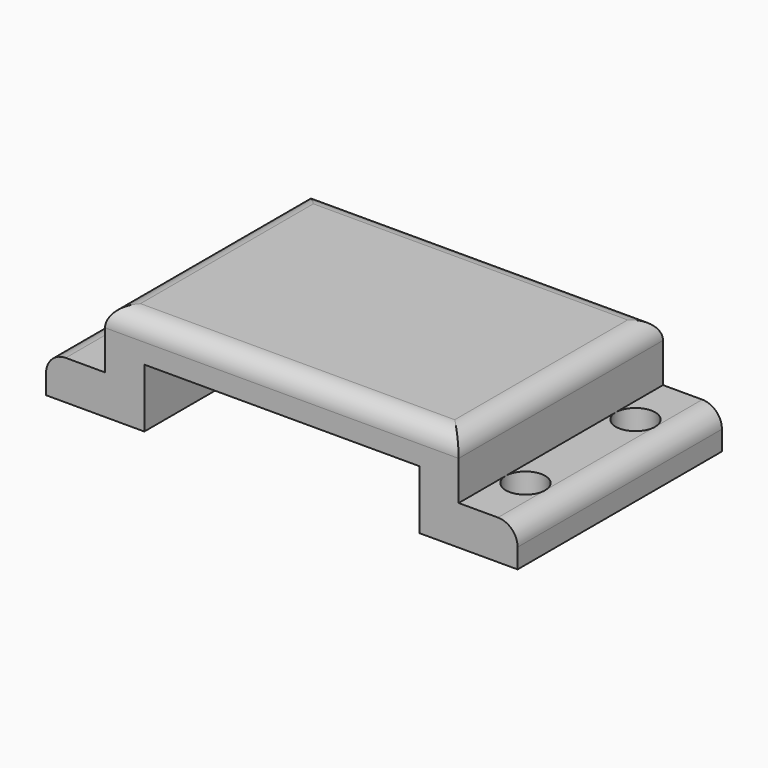
from build123d import *

# Parameters (mm, degrees)
F1_DEPTH = 13
F2_R     = 1
F3_R     = 1
F4_DEPTH = 25
F5_R     = 1
F6_DEPTH = 25


with BuildPart() as f1:
    # F0 (on Front) → F1 (new body)
    with BuildSketch(Plane.XZ):
        Polygon((-20.4238126724, 0), (-18.61380395, 0), (-15.4238126724, 0), (-15.4238126724, 3), (-1.4238126724, 3), (-1.4238126724, 0), (3.5761873276, 0), (3.5761873276, 2), (0.5761873276, 2), (0.5761873276, 5), (-17.4186695367, 5), (-17.4238126724, 2), (-20.4238126724, 2), align=None)
    extrude(amount=F1_DEPTH)

    # F2
    f2_edges = [f1.edges().sort_by_distance(p)[0] for p in [
        (-8.421241, 0, 5),
        (0.576187, -6.5, 5),
        (-17.41867, -6.5, 5),
        (-8.421241, -13, 5),
        (3.576187, -6.5, 2),
        (-20.423813, -6.5, 2),
    ]]
    fillet(f2_edges, radius=F2_R)

    # F3 (on face) → F4 (cut)
    with BuildSketch(Plane(origin=(0, 0, 0), x_dir=(1, 0, 0), z_dir=(0, 0, -1))):
        with Locations((-18.4238126724, 10)):
            Circle(F3_R)
        with Locations((-18.4238126724, 3)):
            Circle(F3_R)
    extrude(amount=-F4_DEPTH, mode=Mode.SUBTRACT)

    # F5 (on face) → F6 (cut)
    with BuildSketch(Plane(origin=(0, 0, 0), x_dir=(1, 0, 0), z_dir=(0, 0, -1))):
        with Locations((1.5761873276, 10)):
            Circle(F5_R)
        with Locations((1.5761873276, 3)):
            Circle(F5_R)
    extrude(amount=-F6_DEPTH, mode=Mode.SUBTRACT)


solid = f1.part
